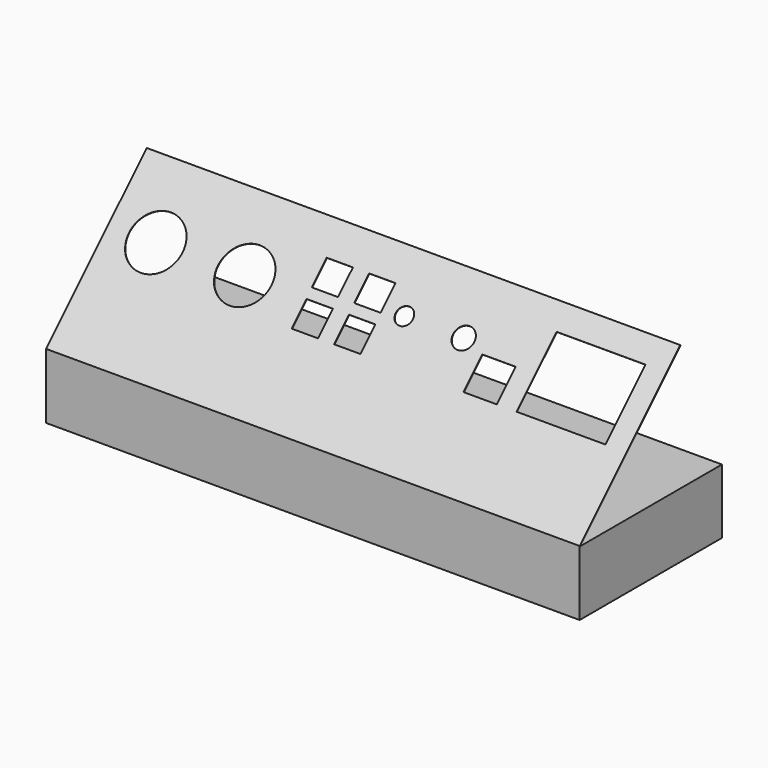
from build123d import *

# Parameters (mm, degrees)
F1_DEPTH = 209.55
F2_W     = 20.6375
F2_H     = 20.6375
F2_W_2   = 20.6374746
F2_W_3   = 69.85
F2_H_2   = 55.5625
F2_W_4   = 26.19375
F2_H_3   = 26.19375
F3_DEPTH = 0.4064


# Not quite as in the source:
# - the dataset's text gives a spline's control points without its knots; the knots are read off the source's solid


with BuildPart() as f1:
    # F0 (on Right) → F1 (new body, symmetric)
    with BuildSketch(Plane.YZ):
        Polygon((-139.7, 0), (0, 0), (0, 50.8), (-139.2936, 50.8), (-139.2936, 51.054), (-40.6298144724, 149.7177855276), (-40.9171826682, 150.0051537235), (-139.7, 51.2223363917), align=None)
    extrude(amount=F1_DEPTH, both=True)

    # F2 (on face) → F3 (cut, through all)
    with BuildSketch(Plane(origin=(0, -95.4611681959, 95.4611681959), x_dir=(1, 0, 0), z_dir=(0, -0.7071067812, 0.7071067812))):
        with Locations((-43.1144662619, 12.8675024964)):
            Rectangle(F2_W, F2_H)
        with Locations((-43.5109856619, 41.4425024964)):
            Rectangle(F2_W, F2_H)
        with Locations((-9.7769662619, 12.8675024964)):
            Rectangle(F2_W, F2_H)
        with Locations((-10.1734983619, 41.4425024964)):
            Rectangle(F2_W_2, F2_H)
        with Locations((158.1011587381, 30.3300024964)):
            Rectangle(F2_W_3, F2_H_2)
        with Locations((94.6011587381, 15.6456274964)):
            Rectangle(F2_W_4, F2_H_3)
        with BuildLine():
            add(Edge.make_bspline(
                [(21.8352387381, 39.0695074964), (20.5863715381, 40.3187048964), (18.8311045381, 41.0456274964), (17.0644329381, 41.0456274964)],
                knots=[7, 7, 7, 7, 8, 8, 8, 8], degree=3))
            add(Edge.make_bspline(
                [(17.0644329381, 41.0456274964), (15.2984979381, 41.0456274964), (13.5432309381, 40.3187048964), (12.2940335381, 39.0695074964)],
                knots=[0, 0, 0, 0, 1, 1, 1, 1], degree=3))
            add(Edge.make_bspline(
                [(12.2940335381, 39.0695074964), (11.0451663381, 37.8209958964), (10.3175579381, 36.0653986964), (10.3175579381, 34.2987524964), (10.3175579381, 32.5327920964), (11.0451663381, 30.7771440964), (12.2940335381, 29.5279720964)],
                knots=[1, 1, 1, 1, 2, 2, 2, 3, 3, 3, 3], degree=3))
            add(Edge.make_bspline(
                [(12.2940335381, 29.5279720964), (13.5432309381, 28.2794858964), (15.2984979381, 27.5518774964), (17.0644329381, 27.5518774964), (18.8311045381, 27.5518774964), (20.5863715381, 28.2794858964), (21.8352387381, 29.5279720964)],
                knots=[3, 3, 3, 3, 4, 4, 4, 5, 5, 5, 5], degree=3))
            add(Edge.make_bspline(
                [(21.8352387381, 29.5279720964), (23.0844107381, 30.7771440964), (23.8113079381, 32.5327920964), (23.8113079381, 34.2987524964), (23.8113079381, 36.0653986964), (23.0844107381, 37.8209958964), (21.8352387381, 39.0695074964)],
                knots=[5, 5, 5, 5, 6, 6, 6, 7, 7, 7, 7], degree=3))
        make_face()
        with BuildLine():
            add(Edge.make_bspline(
                [(-87.3753632619, 38.4569864964), (-91.2690054619, 42.3506286964), (-96.7418418619, 44.6175024964), (-102.2488412619, 44.6175024964)],
                knots=[7, 7, 7, 7, 8, 8, 8, 8], degree=3))
            add(Edge.make_bspline(
                [(-102.2488412619, 44.6175024964), (-107.7551548619, 44.6175024964), (-113.2283468619, 42.3506286964), (-117.1219890619, 38.4569864964)],
                knots=[0, 0, 0, 0, 1, 1, 1, 1], degree=3))
            add(Edge.make_bspline(
                [(-117.1219890619, 38.4569864964), (-121.0156820619, 34.5633442964), (-123.2832162619, 29.0904570964), (-123.2832162619, 23.5831274964), (-123.2832162619, 18.0764836964), (-121.0156820619, 12.6035964964), (-117.1219890619, 8.7092430964)],
                knots=[1, 1, 1, 1, 2, 2, 2, 3, 3, 3, 3], degree=3))
            add(Edge.make_bspline(
                [(-117.1219890619, 8.7092430964), (-113.2283468619, 4.8156008964), (-107.7551548619, 2.5487524964), (-102.2488412619, 2.5487524964), (-96.7418418619, 2.5487524964), (-91.2690054619, 4.8156008964), (-87.3753632619, 8.7092430964)],
                knots=[3, 3, 3, 3, 4, 4, 4, 5, 5, 5, 5], degree=3))
            add(Edge.make_bspline(
                [(-87.3753632619, 8.7092430964), (-83.4813654619, 12.6035964964), (-81.2144662619, 18.0764836964), (-81.2144662619, 23.5831274964), (-81.2144662619, 29.0904570964), (-83.4813654619, 34.5633442964), (-87.3753632619, 38.4569864964)],
                knots=[5, 5, 5, 5, 6, 6, 6, 7, 7, 7, 7], degree=3))
        make_face()
        with BuildLine():
            add(Edge.make_bspline(
                [(-157.2253632619, 38.4569864964), (-161.1190054619, 42.3506286964), (-166.5918418619, 44.6175024964), (-172.0988412619, 44.6175024964)],
                knots=[7, 7, 7, 7, 8, 8, 8, 8], degree=3))
            add(Edge.make_bspline(
                [(-172.0988412619, 44.6175024964), (-177.6051548619, 44.6175024964), (-183.0781690619, 42.3506286964), (-186.9721668619, 38.4569864964), (-190.8661646619, 34.5633442964), (-193.1332162619, 29.0904570964), (-193.1332162619, 23.5831274964), (-193.1332162619, 18.0764836964), (-190.8661646619, 12.6035964964), (-186.9721668619, 8.7092430964)],
                knots=[0, 0, 0, 0, 1, 1, 1, 2, 2, 2, 3, 3, 3, 3], degree=3))
            add(Edge.make_bspline(
                [(-186.9721668619, 8.7092430964), (-183.0781690619, 4.8156008964), (-177.6051548619, 2.5487524964), (-172.0988412619, 2.5487524964), (-166.5918418619, 2.5487524964), (-161.1190054619, 4.8156008964), (-157.2253632619, 8.7092430964)],
                knots=[3, 3, 3, 3, 4, 4, 4, 5, 5, 5, 5], degree=3))
            add(Edge.make_bspline(
                [(-157.2253632619, 8.7092430964), (-153.3313654619, 12.6035964964), (-151.0644662619, 18.0764836964), (-151.0644662619, 23.5831274964), (-151.0644662619, 29.0904570964), (-153.3313654619, 34.5633442964), (-157.2253632619, 38.4569864964)],
                knots=[5, 5, 5, 5, 6, 6, 6, 7, 7, 7, 7], degree=3))
        make_face()
        with BuildLine():
            add(Edge.make_bspline(
                [(69.5828445381, 40.1919080964), (68.0401501381, 41.7353136964), (65.8721585381, 42.6331274964), (63.6896889381, 42.6331274964)],
                knots=[7, 7, 7, 7, 8, 8, 8, 8], degree=3))
            add(Edge.make_bspline(
                [(63.6896889381, 42.6331274964), (61.5075495381, 42.6331274964), (59.3392023381, 41.7353136964), (57.7965079381, 40.1919080964)],
                knots=[0, 0, 0, 0, 1, 1, 1, 1], degree=3))
            add(Edge.make_bspline(
                [(57.7965079381, 40.1919080964), (56.2534579381, 38.6492136964), (55.3553139381, 36.4808664964), (55.3553139381, 34.2987524964), (55.3553139381, 32.1166130964), (56.2534579381, 29.9482658964), (57.7965079381, 28.4055714964)],
                knots=[1, 1, 1, 1, 2, 2, 2, 3, 3, 3, 3], degree=3))
            add(Edge.make_bspline(
                [(57.7965079381, 28.4055714964), (59.3392023381, 26.8628262964), (61.5075495381, 25.9643774964), (63.6896889381, 25.9643774964), (65.8721585381, 25.9643774964), (68.0401501381, 26.8628262964), (69.5828445381, 28.4055714964)],
                knots=[3, 3, 3, 3, 4, 4, 4, 5, 5, 5, 5], degree=3))
            add(Edge.make_bspline(
                [(69.5828445381, 28.4055714964), (71.1259453381, 29.9482658964), (72.0240639381, 32.1166130964), (72.0240639381, 34.2987524964), (72.0240639381, 36.4808664964), (71.1259453381, 38.6492136964), (69.5828445381, 40.1919080964)],
                knots=[5, 5, 5, 5, 6, 6, 6, 7, 7, 7, 7], degree=3))
        make_face()
    extrude(amount=-F3_DEPTH, mode=Mode.SUBTRACT)


solid = f1.part
